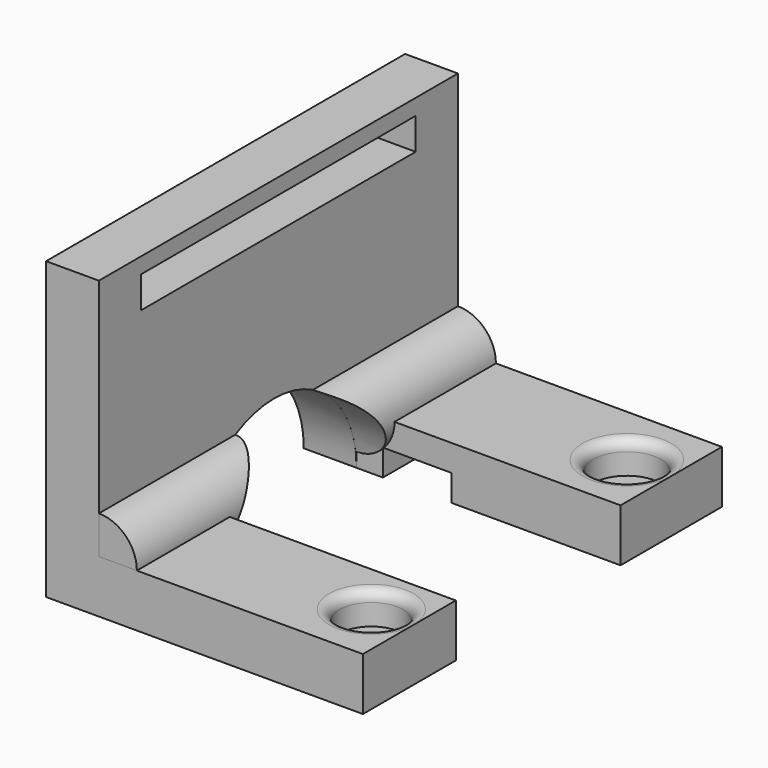
from build123d import *

# Parameters (mm, degrees)
F0_W     = 25
F0_H     = 12
F0_R     = 3.2
F1_DEPTH = 5
F0_H_2   = 11
F0_R_2   = 3
F2_W     = 32.5
F2_H     = 3
F2_W_2   = 12
F2_H_2   = 5
F3_DEPTH = 5
F5_DEPTH = 42.5
F6_W     = 6.5
F6_H     = 6
F7_DEPTH = 2.5
F8_DEPTH = 25
F0_R_3   = 1.6
F9_DEPTH = 2
F0_R_4   = 1.8
F10_R    = 0.99999
F10_2_R  = 0.99999


# Not quite as in the source:
# - a fillet or chamfer is up to 0.001 mm smaller than in the source, because OpenCascade refuses the exact size


with BuildPart() as f1:
    # F0 (on Top) → F1 (new body)
    with BuildSketch(Plane.XY):
        with Locations((-12.5, 36.5)):
            Rectangle(F0_W, F0_H)
        with Locations((-4.2, 36.5)):
            Circle(F0_R, mode=Mode.SUBTRACT)
    extrude(amount=F1_DEPTH)

    # F4 (on face) → F5 (join, through all)
    with BuildSketch(Plane(origin=(0, 42.5, 0), x_dir=(-1, 0, 0), z_dir=(0, 1, 0))):
        with BuildLine():
            Line((25, 1.4033576227), (25, 8.5966423773))
            ThreePointArc((25, 8.5966423773), (21.4033576227, 5), (25, 1.4033576227))
        make_face()
    extrude(amount=-F5_DEPTH)

    # F6 (on face) → F7 (cut)
    with BuildSketch(Plane(origin=(0, 0, 0), x_dir=(1, 0, 0), z_dir=(0, 0, -1))):
        with Locations((-19.25, -33.5)):
            Rectangle(F6_W, F6_H)
    extrude(amount=-F7_DEPTH, mode=Mode.SUBTRACT)

    # F2 (on face) → F8 (cut)
    with BuildSketch(Plane(origin=(-25, 0, 0), x_dir=(0, -1, 0), z_dir=(-1, 0, 0))):
        with BuildLine():
            Line((-30.5, 0), (-11, 0))
            ThreePointArc((-11, 0), (-20.75, 9.75), (-30.5, 0))
        make_face()
    extrude(amount=-F8_DEPTH, mode=Mode.SUBTRACT)

    # F10 (radius 1 in the source; OpenCascade refuses exactly that, so slightly less here)
    f10_edges = [f1.edges().sort_by_distance(p)[0] for p in [
        (-7.4, 36.5, 5),
    ]]
    fillet(f10_edges, radius=F10_R)


with BuildPart() as f1b:
    # F0 (on Top) → F1, piece 2 (new body)
    with BuildSketch(Plane.XY):
        with Locations((-12.5, 5.5)):
            Rectangle(F0_W, F0_H_2)
        with Locations((-4, 6)):
            Circle(F0_R_2, mode=Mode.SUBTRACT)
    extrude(amount=F1_DEPTH)

    # F2 (on face) → F3 (join)
    with BuildSketch(Plane(origin=(-25, 0, 0), x_dir=(0, -1, 0), z_dir=(-1, 0, 0))):
        with BuildLine():
            Line((-11, 0), (0, 0))
            Line((0, 0), (0, 28))
            Line((0, 28), (-42.5, 28))
            Line((-42.5, 28), (-42.5, 5))
            Line((-42.5, 5), (-30.5, 5))
            Line((-30.5, 5), (-30.5, 0))
            ThreePointArc((-30.5, 0), (-20.75, 9.75), (-11, 0))
        make_face()
        with Locations((-21.25, 25)):
            Rectangle(F2_W, F2_H, mode=Mode.SUBTRACT)
        with Locations((-36.5, 2.5)):
            Rectangle(F2_W_2, F2_H_2)
    extrude(amount=F3_DEPTH)

    # F10#2 (radius 1 in the source; OpenCascade refuses exactly that, so slightly less here)
    f10_2_edges = [f1b.edges().sort_by_distance(p)[0] for p in [
        (-7, 6, 5),
    ]]
    fillet(f10_2_edges, radius=F10_2_R)


with BuildPart() as f9:
    # F0 (on Top) → F9 (new body)
    with BuildSketch(Plane.XY):
        with Locations((-4, 6)):
            Circle(F0_R_2)
        with Locations((-4, 6)):
            Circle(F0_R_3, mode=Mode.SUBTRACT)
    extrude(amount=F9_DEPTH)


with BuildPart() as f9b:
    # F0 (on Top) → F9, piece 2 (new body)
    with BuildSketch(Plane.XY):
        with Locations((-4.2, 36.5)):
            Circle(F0_R)
        with Locations((-4.2, 36.5)):
            Circle(F0_R_4, mode=Mode.SUBTRACT)
    extrude(amount=F9_DEPTH)


solid = Compound([f1.part, f1b.part, f9.part, f9b.part])
